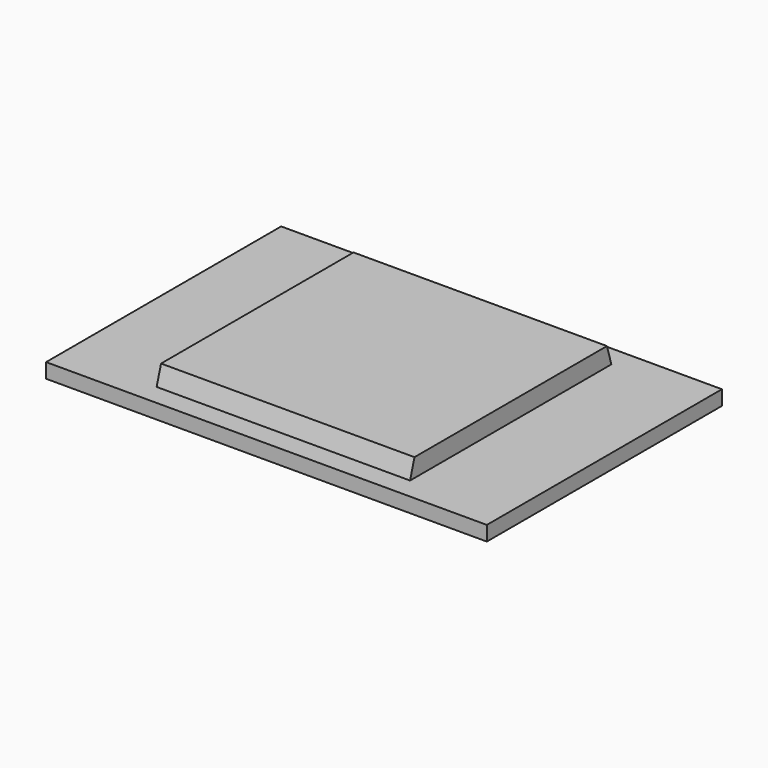
from build123d import *

# Parameters (mm, degrees)
F0_W     = 120
F0_H     = 80
F1_DEPTH = 4
F2_W     = 69
F2_H     = 68.5
F3_DEPTH = 5
F4_SIZE2 = 4.99999
F4_SIZE  = 1.49999


# Not quite as in the source:
# - a fillet or chamfer is up to 0.001 mm smaller than in the source, because OpenCascade refuses the exact size


with BuildPart() as f1:
    # F0 (on Top) → F1 (new body)
    with BuildSketch(Plane.XY):
        Rectangle(F0_W, F0_H)
    extrude(amount=F1_DEPTH)

    # F2 (on face) → F3 (join)
    with BuildSketch(Plane.XY.offset(4)):
        Rectangle(F2_W, F2_H)
    extrude(amount=F3_DEPTH)

    # F4 (size 1.5 and 5 in the source; OpenCascade refuses exactly that, so slightly less here)
    f4_edges = [f1.edges().sort_by_distance(p)[0] for p in [
        (0, 34.25, 9),
        (0, -34.25, 9),
    ]]
    f4_side = f1.faces().sort_by_distance((0, 0, 9))[0]
    chamfer(f4_edges, length=F4_SIZE, length2=F4_SIZE2, reference=f4_side)


solid = f1.part
